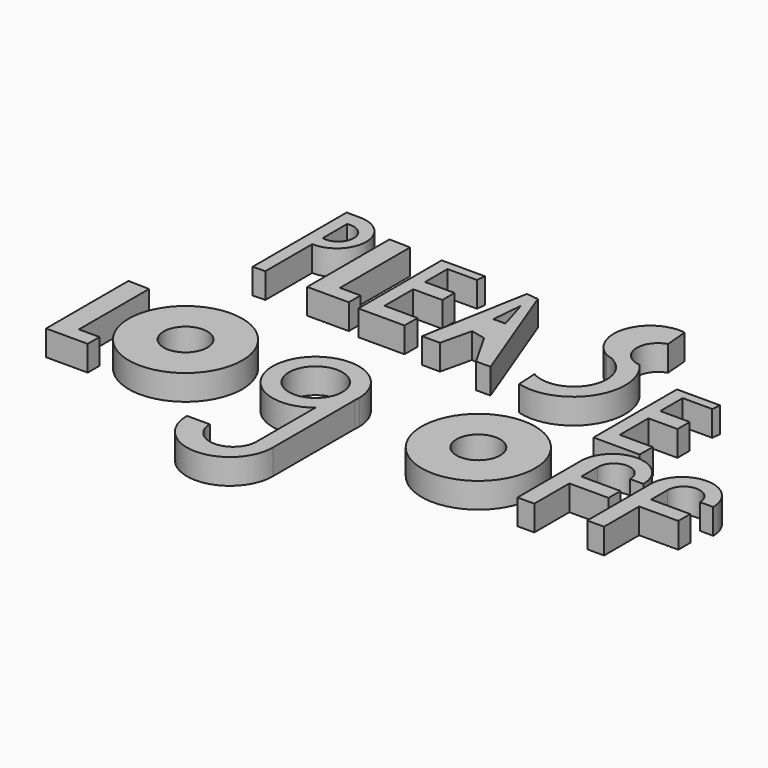
from build123d import *

# Parameters (mm, degrees)
F1_DEPTH = 25.4
F0_R     = 56.8165173198
F0_R_2   = 21.8669462393
F0_R_3   = 26.817322963
F0_W     = 16.8169438839
F0_H     = 43.9109653234
F0_W_2   = 39.239615202
F0_H_2   = 14.948412776
F0_H_3   = 20.5540657043


# Not quite as in the source:
# - a feature names something its author has since deleted; it is built from what else it names


with BuildPart() as f1:
    # F0 (on Top) → F1 (new body)
    with BuildSketch(Plane.XY):
        Polygon((0, 38.4244211018), (-21.0802424699, 38.9997065067), (-21.0802424699, -64.0931278467), (20.6227079034, -64.0931278467), (20.6227079034, -49.3109039962), (0, -49.3109039962), align=None)
    extrude(amount=F1_DEPTH)


with BuildPart() as f1b:
    # F0 (on Top) → F1, piece 2 (new body)
    with BuildSketch(Plane.XY):
        Polygon((-115.4761333019, -144.0774456908), (-136.5563757718, -143.5021602859), (-136.5563757718, -246.5949946394), (-94.8534253985, -246.5949946394), (-94.8534253985, -231.8127707889), (-115.4761333019, -231.8127707889), align=None)
    extrude(amount=F1_DEPTH)


with BuildPart() as f1c:
    # F0 (on Top) → F1, piece 3 (new body)
    with BuildSketch(Plane.XY):
        with BuildLine():
            ThreePointArc((-63.2257908583, -5.0553847104), (-32.6597396912, 24.2578806356), (-63.2257908583, 53.5711459816))
            Line((-63.2257908583, 53.5711459816), (-63.2257908583, 38.5343246162))
            ThreePointArc((-63.2257908583, 38.5343246162), (-44.1613435888, 23.2886993326), (-63.2257908583, 8.0430740491))
            Line((-63.2257908583, 8.0430740491), (-63.2257908583, -5.0553847104))
        make_face()
        Polygon((-63.2257908583, 38.5343246162), (-63.2257908583, 53.5711459816), (-75.7045000792, 53.6349639297), (-75.7045000792, -64.0931278467), (-63.2257908583, -63.6819154024), (-63.2257908583, -5.0553847104), (-63.2257908583, 8.0430740491), align=None)
    extrude(amount=F1_DEPTH)


with BuildPart() as f1d:
    # F0 (on Top) → F1, piece 4 (new body)
    with BuildSketch(Plane.XY):
        Polygon((46.1844839156, -51.2163303792), (46.1844839156, -67.5651431084), (79.0982320905, -67.5651431084), (79.3314799666, -51.2163303792), align=None)
        Polygon((76.328240335, 36.8124432862), (45.7351021469, 36.8124432862), (45.7351021469, 28.0794482678), (75.2847343683, 28.0794482678), align=None)
        Polygon((45.7351021469, 36.8124432862), (32.9688377678, 36.8124432862), (32.9688377678, 0), (45.7351021469, 0), (45.7351021469, 28.0794482678), align=None)
        Polygon((45.7351021469, 0), (32.9688377678, 0), (32.9688377678, -15.3763499111), (46.1844839156, -15.3763499111), (75.2847343683, -15.3763499111), (75.2847343683, 0), align=None)
        Polygon((46.1844839156, -15.3763499111), (32.9688377678, -15.3763499111), (32.9688377678, -67.5651431084), (46.1844839156, -67.5651431084), (46.1844839156, -51.2163303792), align=None)
    extrude(amount=F1_DEPTH)


with BuildPart() as f1e:
    # F0 (on Top) → F1, piece 5 (new body)
    with BuildSketch(Plane.XY):
        Polygon((132.544696331, 32.672625035), (120.5077841878, 34.0194553137), (101.1880040169, -73.1353610754), (119.2409023643, -73.1353610754), (126.4477819204, -41.9589281082), (141.0944137755, -45.3447070969), (160.9281301498, -80.1260992885), (175.3935366869, -80.1260992885), align=None)
        Polygon((138.8186067343, -15.7316308469), (126.7129331827, -15.7316308469), (129.4385045767, 15.4717667028), align=None, mode=Mode.SUBTRACT)
    extrude(amount=F1_DEPTH)


with BuildPart() as f1f:
    # F0 (on Top) → F1, piece 6 (new body)
    with BuildSketch(Plane.XY):
        Polygon((326.3639559736, -107.0016261656), (326.3639559736, -123.3504388947), (359.2777041486, -123.3504388947), (359.5109520247, -107.0016261656), align=None)
        Polygon((356.5077123931, -18.9728525002), (325.9145742049, -18.9728525002), (325.9145742049, -27.7058475185), (355.4642064264, -27.7058475185), align=None)
        Polygon((325.9145742049, -18.9728525002), (313.1483098259, -18.9728525002), (313.1483098259, -55.7852957863), (325.9145742049, -55.7852957863), (325.9145742049, -27.7058475185), align=None)
        Polygon((325.9145742049, -55.7852957863), (313.1483098259, -55.7852957863), (313.1483098259, -71.1616456974), (326.3639559736, -71.1616456974), (355.4642064264, -71.1616456974), (355.4642064264, -55.7852957863), align=None)
        Polygon((326.3639559736, -71.1616456974), (313.1483098259, -71.1616456974), (313.1483098259, -123.3504388947), (326.3639559736, -123.3504388947), (326.3639559736, -107.0016261656), align=None)
    extrude(amount=F1_DEPTH)


with BuildPart() as f1g:
    # F0 (on Top) → F1, piece 7 (new body)
    with BuildSketch(Plane.XY):
        with Locations((-39.7034101188, -193.0736601353)):
            Circle(F0_R)
        with Locations((-39.7034101188, -193.0736601353)):
            Circle(F0_R_2, mode=Mode.SUBTRACT)
    extrude(amount=F1_DEPTH)


with BuildPart() as f1h:
    # F0 (on Top) → F1, piece 8 (new body)
    with BuildSketch(Plane.XY):
        with BuildLine():
            Line((127.9051303864, -293.3522760868), (111.7459100421, -293.3522760868))
            ThreePointArc((111.7459100421, -293.3522760868), (88.3093892006, -316.7887969283), (64.8728683591, -293.3522760868))
            Line((64.8728683591, -293.3522760868), (41.952047497, -293.3522760868))
            ThreePointArc((41.952047497, -293.3522760868), (84.9285889417, -336.3288175315), (127.9051303864, -293.3522760868))
        make_face()
        with BuildLine():
            Line((111.7459100421, -185.910910368), (111.7459100421, -219.7677314667))
            ThreePointArc((111.7459100421, -219.7677314667), (122.8262382091, -206.6285643046), (127.9051303864, -190.208569169))
            Line((127.9051303864, -190.208569169), (127.9051303864, -185.910910368))
            Line((127.9051303864, -185.910910368), (111.7459100421, -185.910910368))
        make_face()
        with BuildLine():
            ThreePointArc((127.9051303864, -190.208569169), (122.8262382091, -206.6285643046), (111.7459100421, -219.7677314667))
            Line((111.7459100421, -219.7677314667), (111.7459100421, -293.3522760868))
            Line((111.7459100421, -293.3522760868), (127.9051303864, -293.3522760868))
            Line((127.9051303864, -293.3522760868), (127.9051303864, -190.208569169))
        make_face()
        with BuildLine():
            ThreePointArc((127.9051303864, -190.208569169), (128.0658585701, -188.0624108039), (128.1194790103, -185.910910368))
            ThreePointArc((128.1194790103, -185.910910368), (46.0459608573, -167.1068011384), (111.7459100421, -219.7677314667))
            Line((111.7459100421, -219.7677314667), (111.7459100421, -185.910910368))
            Line((111.7459100421, -185.910910368), (127.9051303864, -185.910910368))
            Line((127.9051303864, -185.910910368), (127.9051303864, -190.208569169))
        make_face()
        with Locations((84.928587079, -185.910910368)):
            Circle(F0_R_3, mode=Mode.SUBTRACT)
    extrude(amount=F1_DEPTH)


with BuildPart() as f1i:
    # F0 (on Top) → F1, piece 9 (new body)
    with BuildSketch(Plane.XY):
        with Locations((253.241851305, -192.6612166895)):
            Circle(F0_R)
        with Locations((253.241851305, -192.6612166895)):
            Circle(F0_R_2, mode=Mode.SUBTRACT)
    extrude(amount=F1_DEPTH)


with BuildPart() as f1j:
    # F0 (on Top) → F1, piece 10 (new body)
    with BuildSketch(Plane.XY):
        with Locations((338.5631293058, -217.8478464484)):
            Rectangle(F0_W, F0_H)
        with BuildLine():
            ThreePointArc((392.7511572838, -160.3898853064), (361.4529073238, -129.0916353464), (330.1546573639, -160.3898853064))
            Line((330.1546573639, -160.3898853064), (346.9716012478, -160.3898853064))
            ThreePointArc((346.9716012478, -160.3898853064), (363.2073700428, -144.1541165113), (379.4431388378, -160.3898853064))
            Line((379.4431388378, -160.3898853064), (392.7511572838, -160.3898853064))
        make_face()
        with Locations((366.5914088488, -188.4181573987)):
            Rectangle(F0_W_2, F0_H_2)
        with Locations((338.5631293058, -170.6669181585)):
            Rectangle(F0_W, F0_H_3)
        with Locations((338.5631293058, -188.4181573987)):
            Rectangle(F0_W, F0_H_2)
    extrude(amount=F1_DEPTH)


with BuildPart() as f1k:
    # F0 (on Top) → F1, piece 11 (new body)
    with BuildSketch(Plane.XY):
        with Locations((405.560197978, -214.2378575618)):
            Rectangle(F0_W, F0_H)
        with BuildLine():
            ThreePointArc((459.748225956, -156.7798964198), (428.449975996, -125.4816464598), (397.1517260361, -156.7798964198))
            Line((397.1517260361, -156.7798964198), (413.96866992, -156.7798964198))
            ThreePointArc((413.96866992, -156.7798964198), (430.204438715, -140.5441276248), (446.44020751, -156.7798964198))
            Line((446.44020751, -156.7798964198), (459.748225956, -156.7798964198))
        make_face()
        with Locations((433.588477521, -184.8081685121)):
            Rectangle(F0_W_2, F0_H_2)
        with Locations((405.560197978, -167.0569292719)):
            Rectangle(F0_W, F0_H_3)
        with Locations((405.560197978, -184.8081685121)):
            Rectangle(F0_W, F0_H_2)
    extrude(amount=F1_DEPTH)


with BuildPart() as f1l:
    # F0 (on Top) → F1, piece 12 (new body)
    with BuildSketch(Plane.XY):
        with BuildLine():
            Line((259.6997884058, 36.6609323504), (257.7501463465, 60.0499304928))
            ThreePointArc((257.7501463465, 60.0499304928), (217.7821931165, 36.1153467221), (233.6296155648, -7.692880672))
            ThreePointArc((233.6296155648, -7.692880672), (257.4994597468, -51.8785067865), (210.0222513706, -68.2508524094))
            Line((210.0222513706, -68.2508524094), (211.0486635561, -88.7789601735))
            ThreePointArc((211.0486635561, -88.7789601735), (269.1727052446, -66.6322843389), (264.4217915855, -4.6136718735))
            ThreePointArc((264.4217915855, -4.6136718735), (244.806886102, 14.0497048531), (259.6997884058, 36.6609323504))
        make_face()
    extrude(amount=F1_DEPTH)


solid = Compound([f1.part, f1b.part, f1c.part, f1d.part, f1e.part, f1f.part, f1g.part, f1h.part, f1i.part, f1j.part, f1k.part, f1l.part])
